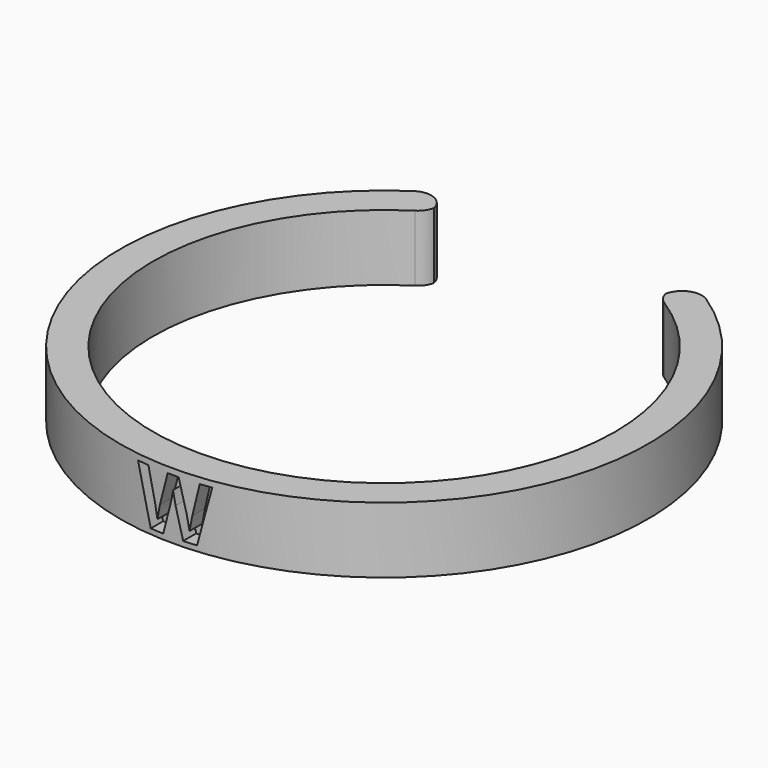
from build123d import *

# Parameters (mm, degrees)
F1_DEPTH     = 10
F0_W         = 15
F0_H         = 1
F2_DEPTH     = 10
F3_TEXT_SIZE = 11.6310767833
F4_DEPTH     = 5
F6_T1_DEPTH  = 18.4260218955
F6_T3_DEPTH  = 36.86169793


# Not quite as in the source:
# - a fillet or chamfer that OpenCascade refuses, or shapes differently, is made with other operations: its cross-section is extruded or revolved along the edge and cut away or added
# - Text() gives the source's letters only with a copy of the font that has no kerning and outlines rounded to 1/6400 em; it was checked with that copy


with BuildPart() as f1:
    # F0 (on Top) → F1 (new body)
    with BuildSketch(Plane.XY):
        with BuildLine():
            ThreePointArc((17.5, 30.3108891325), (30.3108891325, 17.5), (35, 0))
            ThreePointArc((35, 0), (-17.5, -30.3108891325), (-17.5, 30.3108891325))
            Line((-17.5, 30.3108891325), (-17.5, 35.9687364248))
            ThreePointArc((-17.5, 35.9687364248), (-21.2132034356, -33.9116499156), (40, 0))
            ThreePointArc((40, 0), (33.9116499156, 21.2132034356), (17.5, 35.9687364248))
            Line((17.5, 35.9687364248), (17.5, 30.3108891325))
        make_face()
    extrude(amount=F1_DEPTH)


with BuildPart() as f2:
    # F0 (on Top) → F2 (new body)
    with BuildSketch(Plane.XY):
        with Locations((0, -42)):
            Rectangle(F0_W, F0_H)
    extrude(amount=F2_DEPTH)


with BuildPart() as f4_tool:
    # F3 (on face) → F4 (new body)
    with BuildSketch(Plane.XZ.offset(42.5)):
        with Locations((-5.6, 0.812812358)):
            Text('W', F3_TEXT_SIZE, font='Open Sans', font_style=FontStyle.BOLD, text_align=(TextAlign.LEFT, TextAlign.BOTTOM))
    extrude(amount=-F4_DEPTH)


with BuildPart() as f1_1:
    add(f1.part)

    # F4: cut by f4_tool
    add(f4_tool.part, mode=Mode.SUBTRACT)

    # F6: fillet of radius 3 on 4 edges, made by hand

    # F6_s2 → F6_t1 (cut)
    with BuildSketch(Plane.XY.offset(-4.2130109477)):
        with BuildLine():
            ThreePointArc((17.5, 31.9960935116), (17.8679605666, 30.5565212066), (18.8815789474, 29.4700861291))
            ThreePointArc((18.8815789474, 29.4700861291), (18.1956467073, 29.8984688722), (17.5, 30.3108891325))
            Line((17.5, 30.3108891325), (17.5, 31.9960935116))
        make_face()
        with BuildLine():
            ThreePointArc((-17.5, 31.9960935116), (-17.8679605666, 30.5565212066), (-18.8815789474, 29.4700861291))
            ThreePointArc((-18.8815789474, 29.4700861291), (-18.1956467073, 29.8984688722), (-17.5, 30.3108891325))
            Line((-17.5, 30.3108891325), (-17.5, 31.9960935116))
        make_face()
    extrude(amount=F6_T1_DEPTH, mode=Mode.SUBTRACT)

    # F6_s4 → F6_t3 (cut)
    with BuildSketch(Plane.XY.offset(-13.430848965)):
        with BuildLine():
            ThreePointArc((22.1621621622, 33.2992277433), (19.0833995776, 33.4462597583), (17.5, 30.8017856625))
            Line((17.5, 30.8017856625), (17.5, 35.9687364248))
            ThreePointArc((17.5, 35.9687364248), (19.8759489332, 34.7123415229), (22.1621621622, 33.2992277433))
        make_face()
        with BuildLine():
            ThreePointArc((-22.1621621622, 33.2992277433), (-19.0833995776, 33.4462597583), (-17.5, 30.8017856625))
            Line((-17.5, 30.8017856625), (-17.5, 35.9687364248))
            ThreePointArc((-17.5, 35.9687364248), (-19.8759489332, 34.7123415229), (-22.1621621622, 33.2992277433))
        make_face()
    extrude(amount=F6_T3_DEPTH, mode=Mode.SUBTRACT)


with BuildPart() as f2_1:
    add(f2.part)

    # F4: cut by f4_tool
    add(f4_tool.part, mode=Mode.SUBTRACT)


solid = f1_1.part
